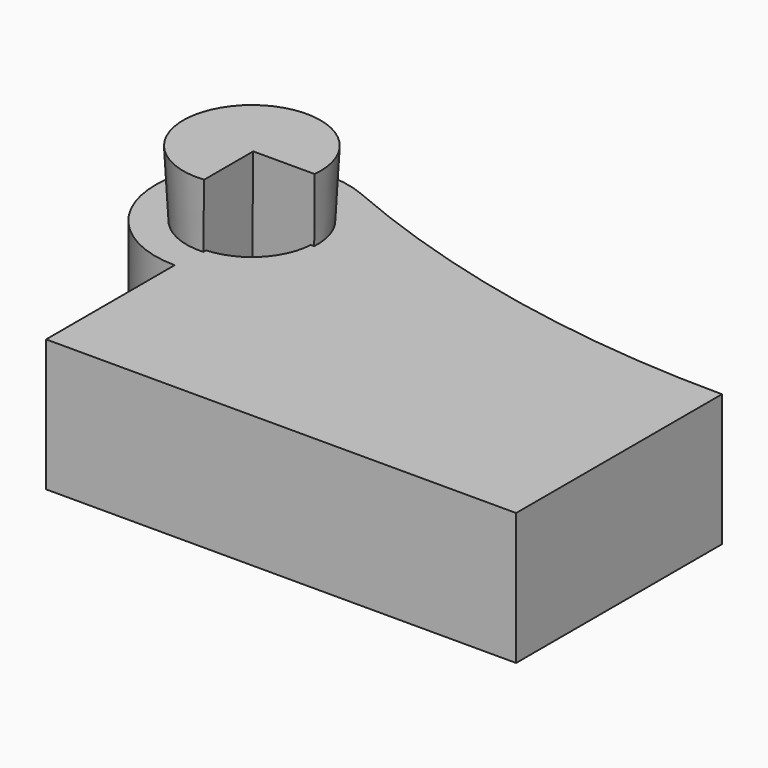
from build123d import *

# Parameters (mm, degrees)
F1_DEPTH               = 12.7
F2_DEPTH               = 25.4
DRAFT_F2_DRAFTED_ANGLE = -3
F3_DEPTH               = 25.4


# Not quite as in the source:
# - an extrude with a draft is written as a straight extrude whose walls are then drafted


with BuildPart() as f1:
    # F0 (on Top) → F1 (new body, symmetric)
    with BuildSketch(Plane.XY):
        with BuildLine():
            ThreePointArc((-37.8976549928, 41.805035811), (-63.3963173264, 28.4760151215), (-45.2116988599, 6.1788353767))
            Line((-45.2116988599, 6.1788353767), (-45.2116988599, 12.8658735537))
            ThreePointArc((-45.2116988599, 12.8658735537), (-53.6098979799, 33.1409197686), (-33.3348517649, 24.7427206486))
            Line((-33.3348517649, 24.7427206486), (-26.647813588, 24.7427206486))
            ThreePointArc((-26.647813588, 24.7427206486), (-29.7133939911, 34.9613498416), (-37.8976549928, 41.805035811))
        make_face()
        with BuildLine():
            Line((-26.647813588, 24.7427206486), (45.2116988599, 24.7427206486))
            ThreePointArc((45.2116988599, 24.7427206486), (2.7903383899, 29.0523227947), (-37.8976549928, 41.805035811))
            ThreePointArc((-37.8976549928, 41.805035811), (-29.7133939911, 34.9613498416), (-26.647813588, 24.7427206486))
        make_face()
        with BuildLine():
            Line((-45.2116988599, -24.7427206486), (45.2116988599, -24.7427206486))
            Line((45.2116988599, -24.7427206486), (45.2116988599, 24.7427206486))
            Line((45.2116988599, 24.7427206486), (-26.647813588, 24.7427206486))
            ThreePointArc((-26.647813588, 24.7427206486), (-32.0850496989, 11.6160714877), (-45.2116988599, 6.1788353767))
            Line((-45.2116988599, 6.1788353767), (-45.2116988599, -24.7427206486))
        make_face()
        with BuildLine():
            Line((-45.2116988599, 12.8658735537), (-45.2116988599, 6.1788353767))
            ThreePointArc((-45.2116988599, 6.1788353767), (-32.0850496989, 11.6160714877), (-26.647813588, 24.7427206486))
            Line((-26.647813588, 24.7427206486), (-33.3348517649, 24.7427206486))
            ThreePointArc((-33.3348517649, 24.7427206486), (-36.8134997399, 16.3445215287), (-45.2116988599, 12.8658735537))
        make_face()
    extrude(amount=F1_DEPTH, both=True)


with BuildPart() as f2_drafted:
    # F0 (on Top) → F2 (new body)
    with BuildSketch(Plane.XY):
        with BuildLine():
            ThreePointArc((-33.3348517649, 24.7427206486), (-53.6098979799, 33.1409197686), (-45.2116988599, 12.8658735537))
            Line((-45.2116988599, 12.8658735537), (-45.2116988599, 24.7427206486))
            Line((-45.2116988599, 24.7427206486), (-33.3348517649, 24.7427206486))
        make_face()
    extrude(amount=F2_DEPTH)

    # draft_F2_drafted
    draft_f2_drafted_walls = [f2_drafted.faces().sort_by_distance(p)[0] for p in [
        (-53.6098979799, 33.1409197686, 16.9333333333),
        (-45.2116988599, 18.8042971012, 16.9333333333),
        (-39.2732753124, 24.7427206486, 16.9333333333),
    ]]
    draft(draft_f2_drafted_walls, neutral_plane=Plane.XY, angle=DRAFT_F2_DRAFTED_ANGLE)


with BuildPart() as f1_1:
    add(f1.part)

    # join_F2_drafted: union F2_drafted
    add(f2_drafted.part)

    # F3 (cut): a face of the model
    f3_faces = [f1_1.faces().sort_by_distance(p)[0] for p in [
        (0, -24.7427206486, 0),
    ]]
    extrude(f3_faces, amount=F3_DEPTH, mode=Mode.SUBTRACT)


solid = f1_1.part
